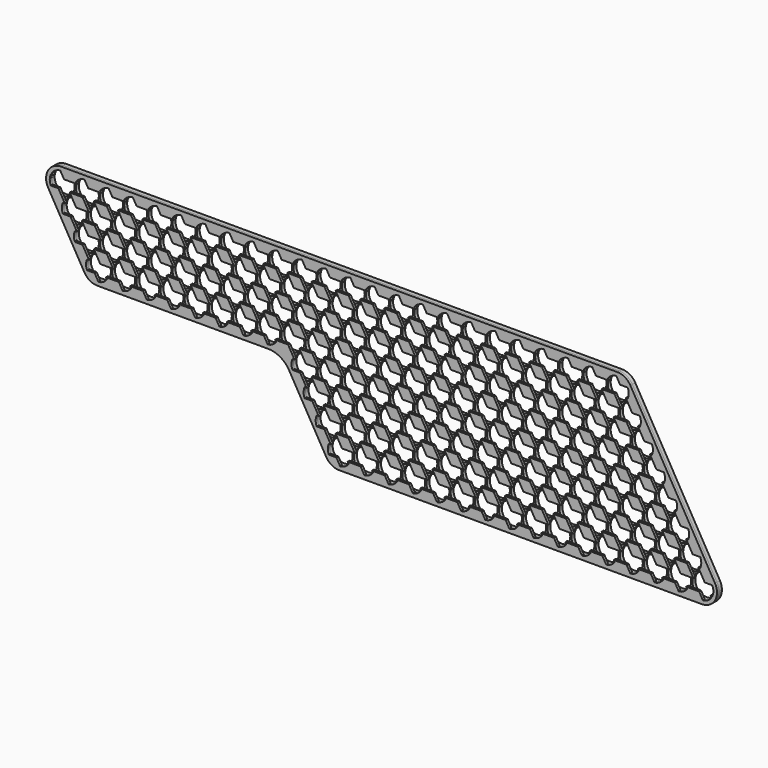
from build123d import *

# Parameters (mm, degrees)
F0_R      = 9.4
F1_DEPTH  = 3
F2_R      = 20
F4_DEPTH  = 2
F6_DEPTH  = 2
F8_DEPTH  = 2
F10_DEPTH = 2
F12_DEPTH = 2


with BuildPart() as f1:
    # F0 (on Front) → F1 (new body)
    with BuildSketch(Plane.XZ):
        with BuildLine():
            ThreePointArc((9.679841755, -7.7498815216), (16.4685048716, -10.4231120583), (19.3, -17.1473029949))
            ThreePointArc((19.3, -17.1473029949), (7.3609322648, -26.1978905469), (1.8716733966, -12.2579296252))
            ThreePointArc((1.8716733966, -12.2579296252), (-5.3694259066, -11.1771760939), (-10.7387150069, -6.2))
            Line((-10.7387150069, -6.2), (18.9612849931, -57.6419089848))
            ThreePointArc((18.9612849931, -57.6419089848), (17.3355686068, -50.5033801767), (20.020158245, -43.6920274632))
            ThreePointArc((20.020158245, -43.6920274632), (13.0758090634, -27.7261011183), (29.2, -34.2946059899))
            ThreePointArc((29.2, -34.2946059899), (28.850587552, -36.833673725), (27.8283266034, -39.1839793596))
            ThreePointArc((27.8283266034, -39.1839793596), (29.7, -39.0419089848), (31.5716733966, -39.1839793596))
            ThreePointArc((31.5716733966, -39.1839793596), (37.0609322648, -25.2440184379), (49, -34.2946059899))
            ThreePointArc((49, -34.2946059899), (46.1685048716, -41.0187969265), (39.379841755, -43.6920274632))
            ThreePointArc((39.379841755, -43.6920274632), (40.4387150069, -45.2419089848), (41.2515151515, -46.9338608812))
            ThreePointArc((41.2515151515, -46.9338608812), (51.8263966154, -42.334336378), (58.9, -51.4419089848))
            ThreePointArc((58.9, -51.4419089848), (51.8263966154, -60.5494815916), (41.2515151515, -55.9499570884))
            ThreePointArc((41.2515151515, -55.9499570884), (36.6950054866, -61.6805562706), (29.7, -63.8419089848))
            Line((29.7, -63.8419089848), (168.3, -63.8419089848))
            ThreePointArc((168.3, -63.8419089848), (161.3049945134, -61.6805562706), (156.7484848485, -55.9499570884))
            ThreePointArc((156.7484848485, -55.9499570884), (139.1, -51.4419089848), (156.7484848485, -46.9338608812))
            ThreePointArc((156.7484848485, -46.9338608812), (157.5612849931, -45.2419089848), (158.620158245, -43.6920274632))
            ThreePointArc((158.620158245, -43.6920274632), (151.6758090634, -27.7261011183), (167.8, -34.2946059899))
            ThreePointArc((167.8, -34.2946059899), (167.450587552, -36.833673725), (166.4283266034, -39.1839793596))
            ThreePointArc((166.4283266034, -39.1839793596), (168.3, -39.0419089848), (170.1716733966, -39.1839793596))
            ThreePointArc((170.1716733966, -39.1839793596), (175.6609322648, -25.2440184379), (187.6, -34.2946059899))
            ThreePointArc((187.6, -34.2946059899), (184.7685048716, -41.0187969265), (177.979841755, -43.6920274632))
            ThreePointArc((177.979841755, -43.6920274632), (179.0387150069, -45.2419089848), (179.8515151515, -46.9338608812))
            ThreePointArc((179.8515151515, -46.9338608812), (190.4263966154, -42.334336378), (197.5, -51.4419089848))
            ThreePointArc((197.5, -51.4419089848), (197.150587552, -53.98097672), (196.1283266034, -56.3312823545))
            ThreePointArc((196.1283266034, -56.3312823545), (198, -56.1892119797), (199.8716733966, -56.3312823545))
            ThreePointArc((199.8716733966, -56.3312823545), (205.3609322648, -42.3913214328), (217.3, -51.4419089848))
            ThreePointArc((217.3, -51.4419089848), (214.4685048716, -58.1660999214), (207.679841755, -60.8393304581))
            ThreePointArc((207.679841755, -60.8393304581), (208.7387150069, -62.3892119797), (209.5515151515, -64.0811638761))
            ThreePointArc((209.5515151515, -64.0811638761), (220.1263966154, -59.4816393729), (227.2, -68.5892119797))
            ThreePointArc((227.2, -68.5892119797), (220.1263966154, -77.6967845865), (209.5515151515, -73.0972600833))
            ThreePointArc((209.5515151515, -73.0972600833), (208.7387150069, -74.7892119797), (207.679841755, -76.3390935013))
            ThreePointArc((207.679841755, -76.3390935013), (214.4685048716, -79.0123240381), (217.3, -85.7365149747))
            ThreePointArc((217.3, -85.7365149747), (205.3609322648, -94.7871025266), (199.8716733966, -80.8471416049))
            ThreePointArc((199.8716733966, -80.8471416049), (192.6305740934, -79.7663880736), (187.2612849931, -74.7892119797))
            Line((187.2612849931, -74.7892119797), (216.9612849931, -126.2311209645))
            ThreePointArc((216.9612849931, -126.2311209645), (215.3355686068, -119.0925921564), (218.020158245, -112.2812394429))
            ThreePointArc((218.020158245, -112.2812394429), (211.0758090634, -96.315313098), (227.2, -102.8838179696))
            ThreePointArc((227.2, -102.8838179696), (226.850587552, -105.4228857048), (225.8283266034, -107.7731913393))
            ThreePointArc((225.8283266034, -107.7731913393), (227.7, -107.6311209645), (229.5716733966, -107.7731913393))
            ThreePointArc((229.5716733966, -107.7731913393), (235.0609322648, -93.8332304176), (247, -102.8838179696))
            ThreePointArc((247, -102.8838179696), (244.1685048716, -109.6080089062), (237.379841755, -112.2812394429))
            ThreePointArc((237.379841755, -112.2812394429), (238.4387150069, -113.8311209645), (239.2515151515, -115.5230728609))
            ThreePointArc((239.2515151515, -115.5230728609), (249.8263966154, -110.9235483577), (256.9, -120.0311209645))
            ThreePointArc((256.9, -120.0311209645), (249.8263966154, -129.1386935713), (239.2515151515, -124.5391690681))
            ThreePointArc((239.2515151515, -124.5391690681), (234.6950054866, -130.2697682503), (227.7, -132.4311209645))
            Line((227.7, -132.4311209645), (524.7, -132.4311209645))
            ThreePointArc((524.7, -132.4311209645), (517.7049945134, -130.2697682503), (513.1484848485, -124.5391690681))
            ThreePointArc((513.1484848485, -124.5391690681), (495.5, -120.0311209645), (513.1484848485, -115.5230728609))
            ThreePointArc((513.1484848485, -115.5230728609), (513.9612849931, -113.8311209645), (515.020158245, -112.2812394429))
            ThreePointArc((515.020158245, -112.2812394429), (508.0758090634, -96.315313098), (524.2, -102.8838179696))
            ThreePointArc((524.2, -102.8838179696), (523.850587552, -105.4228857048), (522.8283266034, -107.7731913393))
            ThreePointArc((522.8283266034, -107.7731913393), (530.0694259066, -108.8539448706), (535.4387150069, -113.8311209645))
            Line((535.4387150069, -113.8311209645), (466.1387150069, 6.2))
            ThreePointArc((466.1387150069, 6.2), (467.377480246, 3.2093561593), (467.8, 0))
            ThreePointArc((467.8, 0), (467.1002144801, -4.1066995409), (465.079841755, -7.7498815216))
            ThreePointArc((465.079841755, -7.7498815216), (471.8685048716, -10.4231120583), (474.7, -17.1473029949))
            ThreePointArc((474.7, -17.1473029949), (462.7609322648, -26.1978905469), (457.2716733966, -12.2579296252))
            ThreePointArc((457.2716733966, -12.2579296252), (455.4, -12.4), (453.5283266034, -12.2579296252))
            ThreePointArc((453.5283266034, -12.2579296252), (454.550587552, -14.6082352597), (454.9, -17.1473029949))
            ThreePointArc((454.9, -17.1473029949), (438.7758090634, -23.7158078665), (445.720158245, -7.7498815216))
            ThreePointArc((445.720158245, -7.7498815216), (444.6612849931, -6.2), (443.8484848485, -4.5080481036))
            ThreePointArc((443.8484848485, -4.5080481036), (426.2, 0), (443.8484848485, 4.5080481036))
            ThreePointArc((443.8484848485, 4.5080481036), (448.4049945134, 10.2386472858), (455.4, 12.4))
            Line((455.4, 12.4), (0, 12.4))
            ThreePointArc((0, 12.4), (6.9950054866, 10.2386472858), (11.5515151515, 4.5080481036))
            ThreePointArc((11.5515151515, 4.5080481036), (22.1263966154, 9.1075726068), (29.2, 0))
            ThreePointArc((29.2, 0), (22.1263966154, -9.1075726068), (11.5515151515, -4.5080481036))
            ThreePointArc((11.5515151515, -4.5080481036), (10.7387150069, -6.2), (9.679841755, -7.7498815216))
        make_face()
        with Locations((257.4, -102.8838179696)):
            Circle(F0_R, mode=Mode.SUBTRACT)
        with Locations((227.7, -85.7365149747)):
            Circle(F0_R, mode=Mode.SUBTRACT)
        with Locations((247.5, -85.7365149747)):
            Circle(F0_R, mode=Mode.SUBTRACT)
        with Locations((237.6, -68.5892119797)):
            Circle(F0_R, mode=Mode.SUBTRACT)
        with Locations((257.4, -68.5892119797)):
            Circle(F0_R, mode=Mode.SUBTRACT)
        with Locations((267.3, -120.0311209645)):
            Circle(F0_R, mode=Mode.SUBTRACT)
        with Locations((287.1, -120.0311209645)):
            Circle(F0_R, mode=Mode.SUBTRACT)
        with Locations((306.9, -120.0311209645)):
            Circle(F0_R, mode=Mode.SUBTRACT)
        with Locations((326.7, -120.0311209645)):
            Circle(F0_R, mode=Mode.SUBTRACT)
        with Locations((346.5, -120.0311209645)):
            Circle(F0_R, mode=Mode.SUBTRACT)
        with Locations((366.3, -120.0311209645)):
            Circle(F0_R, mode=Mode.SUBTRACT)
        with Locations((386.1, -120.0311209645)):
            Circle(F0_R, mode=Mode.SUBTRACT)
        with Locations((277.2, -102.8838179696)):
            Circle(F0_R, mode=Mode.SUBTRACT)
        with Locations((297, -102.8838179696)):
            Circle(F0_R, mode=Mode.SUBTRACT)
        with Locations((316.8, -102.8838179696)):
            Circle(F0_R, mode=Mode.SUBTRACT)
        with Locations((336.6, -102.8838179696)):
            Circle(F0_R, mode=Mode.SUBTRACT)
        with Locations((356.4, -102.8838179696)):
            Circle(F0_R, mode=Mode.SUBTRACT)
        with Locations((376.2, -102.8838179696)):
            Circle(F0_R, mode=Mode.SUBTRACT)
        with Locations((396, -102.8838179696)):
            Circle(F0_R, mode=Mode.SUBTRACT)
        with Locations((405.9, -120.0311209645)):
            Circle(F0_R, mode=Mode.SUBTRACT)
        with Locations((425.7, -120.0311209645)):
            Circle(F0_R, mode=Mode.SUBTRACT)
        with Locations((445.5, -120.0311209645)):
            Circle(F0_R, mode=Mode.SUBTRACT)
        with Locations((465.3, -120.0311209645)):
            Circle(F0_R, mode=Mode.SUBTRACT)
        with Locations((485.1, -120.0311209645)):
            Circle(F0_R, mode=Mode.SUBTRACT)
        with Locations((415.8, -102.8838179696)):
            Circle(F0_R, mode=Mode.SUBTRACT)
        with Locations((435.6, -102.8838179696)):
            Circle(F0_R, mode=Mode.SUBTRACT)
        with Locations((455.4, -102.8838179696)):
            Circle(F0_R, mode=Mode.SUBTRACT)
        with Locations((475.2, -102.8838179696)):
            Circle(F0_R, mode=Mode.SUBTRACT)
        with Locations((495, -102.8838179696)):
            Circle(F0_R, mode=Mode.SUBTRACT)
        with Locations((267.3, -85.7365149747)):
            Circle(F0_R, mode=Mode.SUBTRACT)
        with Locations((287.1, -85.7365149747)):
            Circle(F0_R, mode=Mode.SUBTRACT)
        with Locations((306.9, -85.7365149747)):
            Circle(F0_R, mode=Mode.SUBTRACT)
        with Locations((326.7, -85.7365149747)):
            Circle(F0_R, mode=Mode.SUBTRACT)
        with Locations((346.5, -85.7365149747)):
            Circle(F0_R, mode=Mode.SUBTRACT)
        with Locations((366.3, -85.7365149747)):
            Circle(F0_R, mode=Mode.SUBTRACT)
        with Locations((386.1, -85.7365149747)):
            Circle(F0_R, mode=Mode.SUBTRACT)
        with Locations((277.2, -68.5892119797)):
            Circle(F0_R, mode=Mode.SUBTRACT)
        with Locations((297, -68.5892119797)):
            Circle(F0_R, mode=Mode.SUBTRACT)
        with Locations((316.8, -68.5892119797)):
            Circle(F0_R, mode=Mode.SUBTRACT)
        with Locations((336.6, -68.5892119797)):
            Circle(F0_R, mode=Mode.SUBTRACT)
        with Locations((356.4, -68.5892119797)):
            Circle(F0_R, mode=Mode.SUBTRACT)
        with Locations((376.2, -68.5892119797)):
            Circle(F0_R, mode=Mode.SUBTRACT)
        with Locations((396, -68.5892119797)):
            Circle(F0_R, mode=Mode.SUBTRACT)
        with Locations((405.9, -85.7365149747)):
            Circle(F0_R, mode=Mode.SUBTRACT)
        with Locations((425.7, -85.7365149747)):
            Circle(F0_R, mode=Mode.SUBTRACT)
        with Locations((445.5, -85.7365149747)):
            Circle(F0_R, mode=Mode.SUBTRACT)
        with Locations((465.3, -85.7365149747)):
            Circle(F0_R, mode=Mode.SUBTRACT)
        with Locations((485.1, -85.7365149747)):
            Circle(F0_R, mode=Mode.SUBTRACT)
        with Locations((504.9, -85.7365149747)):
            Circle(F0_R, mode=Mode.SUBTRACT)
        with Locations((415.8, -68.5892119797)):
            Circle(F0_R, mode=Mode.SUBTRACT)
        with Locations((435.6, -68.5892119797)):
            Circle(F0_R, mode=Mode.SUBTRACT)
        with Locations((455.4, -68.5892119797)):
            Circle(F0_R, mode=Mode.SUBTRACT)
        with Locations((475.2, -68.5892119797)):
            Circle(F0_R, mode=Mode.SUBTRACT)
        with Locations((495, -68.5892119797)):
            Circle(F0_R, mode=Mode.SUBTRACT)
        with Locations((69.3, -51.4419089848)):
            Circle(F0_R, mode=Mode.SUBTRACT)
        with Locations((89.1, -51.4419089848)):
            Circle(F0_R, mode=Mode.SUBTRACT)
        with Locations((108.9, -51.4419089848)):
            Circle(F0_R, mode=Mode.SUBTRACT)
        with Locations((59.4, -34.2946059899)):
            Circle(F0_R, mode=Mode.SUBTRACT)
        with Locations((79.2, -34.2946059899)):
            Circle(F0_R, mode=Mode.SUBTRACT)
        with Locations((99, -34.2946059899)):
            Circle(F0_R, mode=Mode.SUBTRACT)
        with Locations((118.8, -34.2946059899)):
            Circle(F0_R, mode=Mode.SUBTRACT)
        with Locations((128.7, -51.4419089848)):
            Circle(F0_R, mode=Mode.SUBTRACT)
        with Locations((227.7, -51.4419089848)):
            Circle(F0_R, mode=Mode.SUBTRACT)
        with Locations((247.5, -51.4419089848)):
            Circle(F0_R, mode=Mode.SUBTRACT)
        with Locations((138.6, -34.2946059899)):
            Circle(F0_R, mode=Mode.SUBTRACT)
        with Locations((198, -34.2946059899)):
            Circle(F0_R, mode=Mode.SUBTRACT)
        with Locations((217.8, -34.2946059899)):
            Circle(F0_R, mode=Mode.SUBTRACT)
        with Locations((237.6, -34.2946059899)):
            Circle(F0_R, mode=Mode.SUBTRACT)
        with Locations((257.4, -34.2946059899)):
            Circle(F0_R, mode=Mode.SUBTRACT)
        with Locations((29.7, -17.1473029949)):
            Circle(F0_R, mode=Mode.SUBTRACT)
        with Locations((49.5, -17.1473029949)):
            Circle(F0_R, mode=Mode.SUBTRACT)
        with Locations((69.3, -17.1473029949)):
            Circle(F0_R, mode=Mode.SUBTRACT)
        with Locations((89.1, -17.1473029949)):
            Circle(F0_R, mode=Mode.SUBTRACT)
        with Locations((108.9, -17.1473029949)):
            Circle(F0_R, mode=Mode.SUBTRACT)
        with Locations((39.6, 0)):
            Circle(F0_R, mode=Mode.SUBTRACT)
        with Locations((59.4, 0)):
            Circle(F0_R, mode=Mode.SUBTRACT)
        with Locations((79.2, 0)):
            Circle(F0_R, mode=Mode.SUBTRACT)
        with Locations((99, 0)):
            Circle(F0_R, mode=Mode.SUBTRACT)
        with Locations((118.8, 0)):
            Circle(F0_R, mode=Mode.SUBTRACT)
        with Locations((128.7, -17.1473029949)):
            Circle(F0_R, mode=Mode.SUBTRACT)
        with Locations((148.5, -17.1473029949)):
            Circle(F0_R, mode=Mode.SUBTRACT)
        with Locations((168.3, -17.1473029949)):
            Circle(F0_R, mode=Mode.SUBTRACT)
        with Locations((188.1, -17.1473029949)):
            Circle(F0_R, mode=Mode.SUBTRACT)
        with Locations((207.9, -17.1473029949)):
            Circle(F0_R, mode=Mode.SUBTRACT)
        with Locations((227.7, -17.1473029949)):
            Circle(F0_R, mode=Mode.SUBTRACT)
        with Locations((247.5, -17.1473029949)):
            Circle(F0_R, mode=Mode.SUBTRACT)
        with Locations((138.6, 0)):
            Circle(F0_R, mode=Mode.SUBTRACT)
        with Locations((158.4, 0)):
            Circle(F0_R, mode=Mode.SUBTRACT)
        with Locations((178.2, 0)):
            Circle(F0_R, mode=Mode.SUBTRACT)
        with Locations((198, 0)):
            Circle(F0_R, mode=Mode.SUBTRACT)
        with Locations((217.8, 0)):
            Circle(F0_R, mode=Mode.SUBTRACT)
        with Locations((237.6, 0)):
            Circle(F0_R, mode=Mode.SUBTRACT)
        with Locations((257.4, 0)):
            Circle(F0_R, mode=Mode.SUBTRACT)
        with Locations((267.3, -51.4419089848)):
            Circle(F0_R, mode=Mode.SUBTRACT)
        with Locations((287.1, -51.4419089848)):
            Circle(F0_R, mode=Mode.SUBTRACT)
        with Locations((306.9, -51.4419089848)):
            Circle(F0_R, mode=Mode.SUBTRACT)
        with Locations((326.7, -51.4419089848)):
            Circle(F0_R, mode=Mode.SUBTRACT)
        with Locations((346.5, -51.4419089848)):
            Circle(F0_R, mode=Mode.SUBTRACT)
        with Locations((366.3, -51.4419089848)):
            Circle(F0_R, mode=Mode.SUBTRACT)
        with Locations((386.1, -51.4419089848)):
            Circle(F0_R, mode=Mode.SUBTRACT)
        with Locations((277.2, -34.2946059899)):
            Circle(F0_R, mode=Mode.SUBTRACT)
        with Locations((297, -34.2946059899)):
            Circle(F0_R, mode=Mode.SUBTRACT)
        with Locations((316.8, -34.2946059899)):
            Circle(F0_R, mode=Mode.SUBTRACT)
        with Locations((336.6, -34.2946059899)):
            Circle(F0_R, mode=Mode.SUBTRACT)
        with Locations((356.4, -34.2946059899)):
            Circle(F0_R, mode=Mode.SUBTRACT)
        with Locations((376.2, -34.2946059899)):
            Circle(F0_R, mode=Mode.SUBTRACT)
        with Locations((396, -34.2946059899)):
            Circle(F0_R, mode=Mode.SUBTRACT)
        with Locations((405.9, -51.4419089848)):
            Circle(F0_R, mode=Mode.SUBTRACT)
        with Locations((425.7, -51.4419089848)):
            Circle(F0_R, mode=Mode.SUBTRACT)
        with Locations((445.5, -51.4419089848)):
            Circle(F0_R, mode=Mode.SUBTRACT)
        with Locations((465.3, -51.4419089848)):
            Circle(F0_R, mode=Mode.SUBTRACT)
        with Locations((485.1, -51.4419089848)):
            Circle(F0_R, mode=Mode.SUBTRACT)
        with Locations((415.8, -34.2946059899)):
            Circle(F0_R, mode=Mode.SUBTRACT)
        with Locations((435.6, -34.2946059899)):
            Circle(F0_R, mode=Mode.SUBTRACT)
        with Locations((455.4, -34.2946059899)):
            Circle(F0_R, mode=Mode.SUBTRACT)
        with Locations((475.2, -34.2946059899)):
            Circle(F0_R, mode=Mode.SUBTRACT)
        with Locations((267.3, -17.1473029949)):
            Circle(F0_R, mode=Mode.SUBTRACT)
        with Locations((287.1, -17.1473029949)):
            Circle(F0_R, mode=Mode.SUBTRACT)
        with Locations((306.9, -17.1473029949)):
            Circle(F0_R, mode=Mode.SUBTRACT)
        with Locations((326.7, -17.1473029949)):
            Circle(F0_R, mode=Mode.SUBTRACT)
        with Locations((346.5, -17.1473029949)):
            Circle(F0_R, mode=Mode.SUBTRACT)
        with Locations((366.3, -17.1473029949)):
            Circle(F0_R, mode=Mode.SUBTRACT)
        with Locations((386.1, -17.1473029949)):
            Circle(F0_R, mode=Mode.SUBTRACT)
        with Locations((277.2, 0)):
            Circle(F0_R, mode=Mode.SUBTRACT)
        with Locations((297, 0)):
            Circle(F0_R, mode=Mode.SUBTRACT)
        with Locations((316.8, 0)):
            Circle(F0_R, mode=Mode.SUBTRACT)
        with Locations((336.6, 0)):
            Circle(F0_R, mode=Mode.SUBTRACT)
        with Locations((356.4, 0)):
            Circle(F0_R, mode=Mode.SUBTRACT)
        with Locations((376.2, 0)):
            Circle(F0_R, mode=Mode.SUBTRACT)
        with Locations((396, 0)):
            Circle(F0_R, mode=Mode.SUBTRACT)
        with Locations((405.9, -17.1473029949)):
            Circle(F0_R, mode=Mode.SUBTRACT)
        with Locations((425.7, -17.1473029949)):
            Circle(F0_R, mode=Mode.SUBTRACT)
        with Locations((415.8, 0)):
            Circle(F0_R, mode=Mode.SUBTRACT)
        with BuildLine():
            ThreePointArc((1.8716733966, -12.2579296252), (5.2, -9.0066641994), (9.679841755, -7.7498815216))
            ThreePointArc((9.679841755, -7.7498815216), (10.7387150069, -6.2), (11.5515151515, -4.5080481036))
            ThreePointArc((11.5515151515, -4.5080481036), (10.4, 0), (11.5515151515, 4.5080481036))
            ThreePointArc((11.5515151515, 4.5080481036), (6.9950054866, 10.2386472858), (0, 12.4))
            ThreePointArc((0, 12.4), (-10.7387150069, 6.2), (-10.7387150069, -6.2))
            ThreePointArc((-10.7387150069, -6.2), (-5.3694259066, -11.1771760939), (1.8716733966, -12.2579296252))
        make_face()
        Circle(F0_R, mode=Mode.SUBTRACT)
        with BuildLine():
            ThreePointArc((20.020158245, -43.6920274632), (17.3355686068, -50.5033801767), (18.9612849931, -57.6419089848))
            ThreePointArc((18.9612849931, -57.6419089848), (23.5, -62.1806239917), (29.7, -63.8419089848))
            ThreePointArc((29.7, -63.8419089848), (36.6950054866, -61.6805562706), (41.2515151515, -55.9499570884))
            ThreePointArc((41.2515151515, -55.9499570884), (40.1, -51.4419089848), (41.2515151515, -46.9338608812))
            ThreePointArc((41.2515151515, -46.9338608812), (40.4387150069, -45.2419089848), (39.379841755, -43.6920274632))
            ThreePointArc((39.379841755, -43.6920274632), (34.9, -42.4352447854), (31.5716733966, -39.1839793596))
            ThreePointArc((31.5716733966, -39.1839793596), (29.7, -39.0419089848), (27.8283266034, -39.1839793596))
            ThreePointArc((27.8283266034, -39.1839793596), (24.5, -42.4352447854), (20.020158245, -43.6920274632))
        make_face()
        with Locations((29.7, -51.4419089848)):
            Circle(F0_R, mode=Mode.SUBTRACT)
        with BuildLine():
            ThreePointArc((466.1387150069, 6.2), (461.6, 10.7387150069), (455.4, 12.4))
            ThreePointArc((455.4, 12.4), (448.4049945134, 10.2386472858), (443.8484848485, 4.5080481036))
            ThreePointArc((443.8484848485, 4.5080481036), (444.7075726068, 2.3263966154), (445, 0))
            ThreePointArc((445, 0), (444.7075726068, -2.3263966154), (443.8484848485, -4.5080481036))
            ThreePointArc((443.8484848485, -4.5080481036), (444.6612849931, -6.2), (445.720158245, -7.7498815216))
            ThreePointArc((445.720158245, -7.7498815216), (450.2, -9.0066641994), (453.5283266034, -12.2579296252))
            ThreePointArc((453.5283266034, -12.2579296252), (455.4, -12.4), (457.2716733966, -12.2579296252))
            ThreePointArc((457.2716733966, -12.2579296252), (460.6, -9.0066641994), (465.079841755, -7.7498815216))
            ThreePointArc((465.079841755, -7.7498815216), (467.1002144801, -4.1066995409), (467.8, 0))
            ThreePointArc((467.8, 0), (467.377480246, 3.2093561593), (466.1387150069, 6.2))
        make_face()
        with Locations((455.4, 0)):
            Circle(F0_R, mode=Mode.SUBTRACT)
        with BuildLine():
            ThreePointArc((156.7484848485, -55.9499570884), (161.3049945134, -61.6805562706), (168.3, -63.8419089848))
            ThreePointArc((168.3, -63.8419089848), (175.2950054866, -61.6805562706), (179.8515151515, -55.9499570884))
            ThreePointArc((179.8515151515, -55.9499570884), (178.7, -51.4419089848), (179.8515151515, -46.9338608812))
            ThreePointArc((179.8515151515, -46.9338608812), (179.0387150069, -45.2419089848), (177.979841755, -43.6920274632))
            ThreePointArc((177.979841755, -43.6920274632), (173.5, -42.4352447854), (170.1716733966, -39.1839793596))
            ThreePointArc((170.1716733966, -39.1839793596), (168.3, -39.0419089848), (166.4283266034, -39.1839793596))
            ThreePointArc((166.4283266034, -39.1839793596), (163.1, -42.4352447854), (158.620158245, -43.6920274632))
            ThreePointArc((158.620158245, -43.6920274632), (157.5612849931, -45.2419089848), (156.7484848485, -46.9338608812))
            ThreePointArc((156.7484848485, -46.9338608812), (157.6075726068, -49.1155123694), (157.9, -51.4419089848))
            ThreePointArc((157.9, -51.4419089848), (157.6075726068, -53.7683056002), (156.7484848485, -55.9499570884))
        make_face()
        with Locations((168.3, -51.4419089848)):
            Circle(F0_R, mode=Mode.SUBTRACT)
        with BuildLine():
            ThreePointArc((179.8515151515, -55.9499570884), (175.2950054866, -61.6805562706), (168.3, -63.8419089848))
            Line((168.3, -63.8419089848), (180.940856662, -63.8419089848))
            Line((180.940856662, -63.8419089848), (187.2612849931, -74.7892119797))
            ThreePointArc((187.2612849931, -74.7892119797), (185.6355686068, -67.6506831716), (188.320158245, -60.8393304581))
            ThreePointArc((188.320158245, -60.8393304581), (183.4, -59.5825477804), (179.8515151515, -55.9499570884))
        make_face()
        with BuildLine():
            ThreePointArc((537.1, -120.0311209645), (536.677480246, -116.8217648053), (535.4387150069, -113.8311209645))
            ThreePointArc((535.4387150069, -113.8311209645), (530.0694259066, -108.8539448706), (522.8283266034, -107.7731913393))
            ThreePointArc((522.8283266034, -107.7731913393), (519.5, -111.0244567652), (515.020158245, -112.2812394429))
            ThreePointArc((515.020158245, -112.2812394429), (513.9612849931, -113.8311209645), (513.1484848485, -115.5230728609))
            ThreePointArc((513.1484848485, -115.5230728609), (514.0075726068, -117.7047243491), (514.3, -120.0311209645))
            ThreePointArc((514.3, -120.0311209645), (514.0075726068, -122.3575175799), (513.1484848485, -124.5391690681))
            ThreePointArc((513.1484848485, -124.5391690681), (517.7049945134, -130.2697682503), (524.7, -132.4311209645))
            ThreePointArc((524.7, -132.4311209645), (533.4681240867, -128.7992450512), (537.1, -120.0311209645))
        make_face()
        with Locations((524.7, -120.0311209645)):
            Circle(F0_R, mode=Mode.SUBTRACT)
        with BuildLine():
            ThreePointArc((196.1283266034, -56.3312823545), (192.8, -59.5825477804), (188.320158245, -60.8393304581))
            ThreePointArc((188.320158245, -60.8393304581), (185.6355686068, -67.6506831716), (187.2612849931, -74.7892119797))
            ThreePointArc((187.2612849931, -74.7892119797), (192.6305740934, -79.7663880736), (199.8716733966, -80.8471416049))
            ThreePointArc((199.8716733966, -80.8471416049), (203.2, -77.5958761791), (207.679841755, -76.3390935013))
            ThreePointArc((207.679841755, -76.3390935013), (208.7387150069, -74.7892119797), (209.5515151515, -73.0972600833))
            ThreePointArc((209.5515151515, -73.0972600833), (208.4, -68.5892119797), (209.5515151515, -64.0811638761))
            ThreePointArc((209.5515151515, -64.0811638761), (208.7387150069, -62.3892119797), (207.679841755, -60.8393304581))
            ThreePointArc((207.679841755, -60.8393304581), (203.2, -59.5825477804), (199.8716733966, -56.3312823545))
            ThreePointArc((199.8716733966, -56.3312823545), (198, -56.1892119797), (196.1283266034, -56.3312823545))
        make_face()
        with Locations((198, -68.5892119797)):
            Circle(F0_R, mode=Mode.SUBTRACT)
        with BuildLine():
            ThreePointArc((218.020158245, -112.2812394429), (215.3355686068, -119.0925921564), (216.9612849931, -126.2311209645))
            ThreePointArc((216.9612849931, -126.2311209645), (221.5, -130.7698359715), (227.7, -132.4311209645))
            ThreePointArc((227.7, -132.4311209645), (234.6950054866, -130.2697682503), (239.2515151515, -124.5391690681))
            ThreePointArc((239.2515151515, -124.5391690681), (238.1, -120.0311209645), (239.2515151515, -115.5230728609))
            ThreePointArc((239.2515151515, -115.5230728609), (238.4387150069, -113.8311209645), (237.379841755, -112.2812394429))
            ThreePointArc((237.379841755, -112.2812394429), (232.9, -111.0244567652), (229.5716733966, -107.7731913393))
            ThreePointArc((229.5716733966, -107.7731913393), (227.7, -107.6311209645), (225.8283266034, -107.7731913393))
            ThreePointArc((225.8283266034, -107.7731913393), (222.5, -111.0244567652), (218.020158245, -112.2812394429))
        make_face()
        with Locations((227.7, -120.0311209645)):
            Circle(F0_R, mode=Mode.SUBTRACT)
    extrude(amount=F1_DEPTH)

    # F2
    f2_edges = [f1.edges().sort_by_distance(p)[0] for p in [
        (180.940857, -1.5, -63.841909),
    ]]
    fillet(f2_edges, radius=F2_R)


with BuildPart() as f4:
    # F3 (on face) → F4 (new body)
    with BuildSketch(Plane.XZ.offset(3)):
        with BuildLine():
            ThreePointArc((466.1387150069, 6.2), (461.6, 10.7387150069), (455.4, 12.4))
            Line((455.4, 12.4), (0, 12.4))
            ThreePointArc((0, 12.4), (-10.7387150069, 6.2), (-10.7387150069, -6.2))
            Line((-10.7387150069, -6.2), (18.9612849931, -57.6419089848))
            ThreePointArc((18.9612849931, -57.6419089848), (23.5, -62.1806239917), (29.7, -63.8419089848))
            Line((29.7, -63.8419089848), (169.3938512783, -63.8419089848))
            ThreePointArc((169.3938512783, -63.8419089848), (179.3938512783, -66.5214009091), (186.7143593539, -73.8419089848))
            Line((186.7143593539, -73.8419089848), (216.9612849931, -126.2311209645))
            ThreePointArc((216.9612849931, -126.2311209645), (221.5, -130.7698359715), (227.7, -132.4311209645))
            Line((227.7, -132.4311209645), (524.7, -132.4311209645))
            ThreePointArc((524.7, -132.4311209645), (535.4387150069, -126.2311209645), (535.4387150069, -113.8311209645))
            Line((535.4387150069, -113.8311209645), (466.1387150069, 6.2))
        make_face()
    extrude(amount=F4_DEPTH)

    # F5 (on face) → F6 (cut, through all)
    with BuildSketch(Plane.XZ.offset(3)):
        with BuildLine():
            Line((0, 4), (-8.5064681273, 4))
            ThreePointArc((-8.5064681273, 4), (-9.4, 0), (-8.5064681273, -4))
            Line((-8.5064681273, -4), (0, -4))
            Line((0, -4), (463.9064681273, -4))
            ThreePointArc((463.9064681273, -4), (464.8, 0), (463.9064681273, 4))
            Line((463.9064681273, 4), (0, 4))
        make_face()
        with BuildLine():
            Line((29.7, -47.4419089848), (21.1935318727, -47.4419089848))
            ThreePointArc((21.1935318727, -47.4419089848), (20.3, -51.4419089848), (21.1935318727, -55.4419089848))
            Line((21.1935318727, -55.4419089848), (29.7, -55.4419089848))
            Line((29.7, -55.4419089848), (493.6064681273, -55.4419089848))
            ThreePointArc((493.6064681273, -55.4419089848), (494.5, -51.4419089848), (493.6064681273, -47.4419089848))
            Line((493.6064681273, -47.4419089848), (29.7, -47.4419089848))
        make_face()
        with BuildLine():
            Line((9.9, -13.1473029949), (1.3935318727, -13.1473029949))
            ThreePointArc((1.3935318727, -13.1473029949), (0.5, -17.1473029949), (1.3935318727, -21.1473029949))
            Line((1.3935318727, -21.1473029949), (9.9, -21.1473029949))
            Line((9.9, -21.1473029949), (473.8064681273, -21.1473029949))
            ThreePointArc((473.8064681273, -21.1473029949), (474.7, -17.1473029949), (473.8064681273, -13.1473029949))
            Line((473.8064681273, -13.1473029949), (9.9, -13.1473029949))
        make_face()
        with BuildLine():
            Line((19.8, -30.2946059899), (11.2935318727, -30.2946059899))
            ThreePointArc((11.2935318727, -30.2946059899), (10.4, -34.2946059899), (11.2935318727, -38.2946059899))
            Line((11.2935318727, -38.2946059899), (19.8, -38.2946059899))
            Line((19.8, -38.2946059899), (483.7064681273, -38.2946059899))
            ThreePointArc((483.7064681273, -38.2946059899), (484.6, -34.2946059899), (483.7064681273, -30.2946059899))
            Line((483.7064681273, -30.2946059899), (19.8, -30.2946059899))
        make_face()
    extrude(amount=F6_DEPTH, mode=Mode.SUBTRACT)

    # F7 (on face) → F8 (cut, through all)
    with BuildSketch(Plane.XZ.offset(3)):
        with BuildLine():
            Line((198, -64.5892119797), (189.4935318727, -64.5892119797))
            ThreePointArc((189.4935318727, -64.5892119797), (188.6, -68.5892119797), (189.4935318727, -72.5892119797))
            Line((189.4935318727, -72.5892119797), (198, -72.5892119797))
            Line((198, -72.5892119797), (495, -72.5892119797))
            Line((495, -72.5892119797), (503.5064681273, -72.5892119797))
            ThreePointArc((503.5064681273, -72.5892119797), (504.4, -68.5892119797), (503.5064681273, -64.5892119797))
            Line((503.5064681273, -64.5892119797), (495, -64.5892119797))
            Line((495, -64.5892119797), (198, -64.5892119797))
        make_face()
        with BuildLine():
            Line((227.7, -116.0311209645), (219.1935318727, -116.0311209645))
            ThreePointArc((219.1935318727, -116.0311209645), (218.3, -120.0311209645), (219.1935318727, -124.0311209645))
            Line((219.1935318727, -124.0311209645), (227.7, -124.0311209645))
            Line((227.7, -124.0311209645), (524.7, -124.0311209645))
            Line((524.7, -124.0311209645), (533.2064681273, -124.0311209645))
            ThreePointArc((533.2064681273, -124.0311209645), (534.1, -120.0311209645), (533.2064681273, -116.0311209645))
            Line((533.2064681273, -116.0311209645), (524.7, -116.0311209645))
            Line((524.7, -116.0311209645), (227.7, -116.0311209645))
        make_face()
        with BuildLine():
            Line((207.9, -81.7365149747), (199.3935318727, -81.7365149747))
            ThreePointArc((199.3935318727, -81.7365149747), (198.5, -85.7365149747), (199.3935318727, -89.7365149747))
            Line((199.3935318727, -89.7365149747), (207.9, -89.7365149747))
            Line((207.9, -89.7365149747), (504.9, -89.7365149747))
            Line((504.9, -89.7365149747), (513.4064681273, -89.7365149747))
            ThreePointArc((513.4064681273, -89.7365149747), (514.3, -85.7365149747), (513.4064681273, -81.7365149747))
            Line((513.4064681273, -81.7365149747), (504.9, -81.7365149747))
            Line((504.9, -81.7365149747), (207.9, -81.7365149747))
        make_face()
        with BuildLine():
            Line((217.8, -98.8838179696), (209.2935318727, -98.8838179696))
            ThreePointArc((209.2935318727, -98.8838179696), (208.4, -102.8838179696), (209.2935318727, -106.8838179696))
            Line((209.2935318727, -106.8838179696), (217.8, -106.8838179696))
            Line((217.8, -106.8838179696), (514.8, -106.8838179696))
            Line((514.8, -106.8838179696), (523.3064681273, -106.8838179696))
            ThreePointArc((523.3064681273, -106.8838179696), (524.2, -102.8838179696), (523.3064681273, -98.8838179696))
            Line((523.3064681273, -98.8838179696), (514.8, -98.8838179696))
            Line((514.8, -98.8838179696), (217.8, -98.8838179696))
        make_face()
    extrude(amount=F8_DEPTH, mode=Mode.SUBTRACT)

    # F9 (on face) → F10 (cut, through all)
    with BuildSketch(Plane.XZ.offset(3)):
        with BuildLine():
            Line((3.4641016151, 2), (-0.7891324485, 9.3668174947))
            ThreePointArc((-0.7891324485, 9.3668174947), (-4.7, 8.1406387956), (-7.7173356788, 5.3668174947))
            Line((-7.7173356788, 5.3668174947), (-3.4641016151, -2))
            Line((-3.4641016151, -2), (26.2358983849, -53.4419089848))
            Line((26.2358983849, -53.4419089848), (30.4891324485, -60.8087264795))
            ThreePointArc((30.4891324485, -60.8087264795), (34.4, -59.5825477804), (37.4173356788, -56.8087264795))
            Line((37.4173356788, -56.8087264795), (33.1641016151, -49.4419089848))
            Line((33.1641016151, -49.4419089848), (3.4641016151, 2))
        make_face()
        with BuildLine():
            Line((23.2641016151, 2), (19.0108675515, 9.3668174947))
            ThreePointArc((19.0108675515, 9.3668174947), (15.1, 8.1406387956), (12.0826643212, 5.3668174947))
            Line((12.0826643212, 5.3668174947), (16.3358983849, -2))
            Line((16.3358983849, -2), (46.0358983849, -53.4419089848))
            Line((46.0358983849, -53.4419089848), (50.2891324485, -60.8087264795))
            ThreePointArc((50.2891324485, -60.8087264795), (54.2, -59.5825477804), (57.2173356788, -56.8087264795))
            Line((57.2173356788, -56.8087264795), (52.9641016151, -49.4419089848))
            Line((52.9641016151, -49.4419089848), (23.2641016151, 2))
        make_face()
        with BuildLine():
            Line((43.0641016151, 2), (38.8108675515, 9.3668174947))
            ThreePointArc((38.8108675515, 9.3668174947), (34.9, 8.1406387956), (31.8826643212, 5.3668174947))
            Line((31.8826643212, 5.3668174947), (36.1358983849, -2))
            Line((36.1358983849, -2), (65.8358983849, -53.4419089848))
            Line((65.8358983849, -53.4419089848), (70.0891324485, -60.8087264795))
            ThreePointArc((70.0891324485, -60.8087264795), (74, -59.5825477804), (77.0173356788, -56.8087264795))
            Line((77.0173356788, -56.8087264795), (72.7641016151, -49.4419089848))
            Line((72.7641016151, -49.4419089848), (43.0641016151, 2))
        make_face()
        with BuildLine():
            Line((62.8641016151, 2), (58.6108675515, 9.3668174947))
            ThreePointArc((58.6108675515, 9.3668174947), (54.7, 8.1406387956), (51.6826643212, 5.3668174947))
            Line((51.6826643212, 5.3668174947), (55.9358983849, -2))
            Line((55.9358983849, -2), (85.6358983849, -53.4419089848))
            Line((85.6358983849, -53.4419089848), (89.8891324485, -60.8087264795))
            ThreePointArc((89.8891324485, -60.8087264795), (93.8, -59.5825477804), (96.8173356788, -56.8087264795))
            Line((96.8173356788, -56.8087264795), (92.5641016151, -49.4419089848))
            Line((92.5641016151, -49.4419089848), (62.8641016151, 2))
        make_face()
        with BuildLine():
            Line((82.6641016151, 2), (78.4108675515, 9.3668174947))
            ThreePointArc((78.4108675515, 9.3668174947), (74.5, 8.1406387956), (71.4826643212, 5.3668174947))
            Line((71.4826643212, 5.3668174947), (75.7358983849, -2))
            Line((75.7358983849, -2), (105.4358983849, -53.4419089848))
            Line((105.4358983849, -53.4419089848), (109.6891324485, -60.8087264795))
            ThreePointArc((109.6891324485, -60.8087264795), (113.6, -59.5825477804), (116.6173356788, -56.8087264795))
            Line((116.6173356788, -56.8087264795), (112.3641016151, -49.4419089848))
            Line((112.3641016151, -49.4419089848), (82.6641016151, 2))
        make_face()
        with BuildLine():
            Line((102.4641016151, 2), (98.2108675515, 9.3668174947))
            ThreePointArc((98.2108675515, 9.3668174947), (94.3, 8.1406387956), (91.2826643212, 5.3668174947))
            Line((91.2826643212, 5.3668174947), (95.5358983849, -2))
            Line((95.5358983849, -2), (125.2358983849, -53.4419089848))
            Line((125.2358983849, -53.4419089848), (129.4891324485, -60.8087264795))
            ThreePointArc((129.4891324485, -60.8087264795), (133.4, -59.5825477804), (136.4173356788, -56.8087264795))
            Line((136.4173356788, -56.8087264795), (132.1641016151, -49.4419089848))
            Line((132.1641016151, -49.4419089848), (102.4641016151, 2))
        make_face()
        with BuildLine():
            Line((122.2641016151, 2), (118.0108675515, 9.3668174947))
            ThreePointArc((118.0108675515, 9.3668174947), (114.1, 8.1406387956), (111.0826643212, 5.3668174947))
            Line((111.0826643212, 5.3668174947), (115.3358983849, -2))
            Line((115.3358983849, -2), (145.0358983849, -53.4419089848))
            Line((145.0358983849, -53.4419089848), (149.2891324485, -60.8087264795))
            ThreePointArc((149.2891324485, -60.8087264795), (153.2, -59.5825477804), (156.2173356788, -56.8087264795))
            Line((156.2173356788, -56.8087264795), (151.9641016151, -49.4419089848))
            Line((151.9641016151, -49.4419089848), (122.2641016151, 2))
        make_face()
        with BuildLine():
            Line((142.0641016151, 2), (137.8108675515, 9.3668174947))
            ThreePointArc((137.8108675515, 9.3668174947), (133.9, 8.1406387956), (130.8826643212, 5.3668174947))
            Line((130.8826643212, 5.3668174947), (135.1358983849, -2))
            Line((135.1358983849, -2), (164.8358983849, -53.4419089848))
            Line((164.8358983849, -53.4419089848), (169.0891324485, -60.8087264795))
            ThreePointArc((169.0891324485, -60.8087264795), (173, -59.5825477804), (176.0173356788, -56.8087264795))
            Line((176.0173356788, -56.8087264795), (171.7641016151, -49.4419089848))
            Line((171.7641016151, -49.4419089848), (142.0641016151, 2))
        make_face()
    extrude(amount=F10_DEPTH, mode=Mode.SUBTRACT)

    # F11 (on face) → F12 (cut, through all)
    with BuildSketch(Plane.XZ.offset(3)):
        with BuildLine():
            Line((161.8641016151, 2), (157.6108675515, 9.3668174947))
            ThreePointArc((157.6108675515, 9.3668174947), (153.7, 8.1406387956), (150.6826643212, 5.3668174947))
            Line((150.6826643212, 5.3668174947), (154.9358983849, -2))
            Line((154.9358983849, -2), (224.2358983849, -122.0311209645))
            Line((224.2358983849, -122.0311209645), (228.4891324485, -129.3979384592))
            ThreePointArc((228.4891324485, -129.3979384592), (232.4, -128.1717597601), (235.4173356788, -125.3979384592))
            Line((235.4173356788, -125.3979384592), (231.1641016151, -118.0311209645))
            Line((231.1641016151, -118.0311209645), (161.8641016151, 2))
        make_face()
        with BuildLine():
            Line((181.6641016151, 2), (177.4108675515, 9.3668174947))
            ThreePointArc((177.4108675515, 9.3668174947), (173.5, 8.1406387956), (170.4826643212, 5.3668174947))
            Line((170.4826643212, 5.3668174947), (174.7358983849, -2))
            Line((174.7358983849, -2), (244.0358983849, -122.0311209645))
            Line((244.0358983849, -122.0311209645), (248.2891324485, -129.3979384592))
            ThreePointArc((248.2891324485, -129.3979384592), (252.2, -128.1717597601), (255.2173356788, -125.3979384592))
            Line((255.2173356788, -125.3979384592), (250.9641016151, -118.0311209645))
            Line((250.9641016151, -118.0311209645), (181.6641016151, 2))
        make_face()
        with BuildLine():
            Line((201.4641016151, 2), (197.2108675515, 9.3668174947))
            ThreePointArc((197.2108675515, 9.3668174947), (193.3, 8.1406387956), (190.2826643212, 5.3668174947))
            Line((190.2826643212, 5.3668174947), (194.5358983849, -2))
            Line((194.5358983849, -2), (263.8358983849, -122.0311209645))
            Line((263.8358983849, -122.0311209645), (268.0891324485, -129.3979384592))
            ThreePointArc((268.0891324485, -129.3979384592), (272, -128.1717597601), (275.0173356788, -125.3979384592))
            Line((275.0173356788, -125.3979384592), (270.7641016151, -118.0311209645))
            Line((270.7641016151, -118.0311209645), (201.4641016151, 2))
        make_face()
        with BuildLine():
            Line((221.2641016151, 2), (217.0108675515, 9.3668174947))
            ThreePointArc((217.0108675515, 9.3668174947), (213.1, 8.1406387956), (210.0826643212, 5.3668174947))
            Line((210.0826643212, 5.3668174947), (214.3358983849, -2))
            Line((214.3358983849, -2), (283.6358983849, -122.0311209645))
            Line((283.6358983849, -122.0311209645), (287.8891324485, -129.3979384592))
            ThreePointArc((287.8891324485, -129.3979384592), (291.8, -128.1717597601), (294.8173356788, -125.3979384592))
            Line((294.8173356788, -125.3979384592), (290.5641016151, -118.0311209645))
            Line((290.5641016151, -118.0311209645), (221.2641016151, 2))
        make_face()
        with BuildLine():
            Line((241.0641016151, 2), (236.8108675515, 9.3668174947))
            ThreePointArc((236.8108675515, 9.3668174947), (232.9, 8.1406387956), (229.8826643212, 5.3668174947))
            Line((229.8826643212, 5.3668174947), (234.1358983849, -2))
            Line((234.1358983849, -2), (303.4358983849, -122.0311209645))
            Line((303.4358983849, -122.0311209645), (307.6891324485, -129.3979384592))
            ThreePointArc((307.6891324485, -129.3979384592), (311.6, -128.1717597601), (314.6173356788, -125.3979384592))
            Line((314.6173356788, -125.3979384592), (310.3641016151, -118.0311209645))
            Line((310.3641016151, -118.0311209645), (241.0641016151, 2))
        make_face()
        with BuildLine():
            Line((260.8641016151, 2), (256.6108675515, 9.3668174947))
            ThreePointArc((256.6108675515, 9.3668174947), (252.7, 8.1406387956), (249.6826643212, 5.3668174947))
            Line((249.6826643212, 5.3668174947), (253.9358983849, -2))
            Line((253.9358983849, -2), (323.2358983849, -122.0311209645))
            Line((323.2358983849, -122.0311209645), (327.4891324485, -129.3979384592))
            ThreePointArc((327.4891324485, -129.3979384592), (331.4, -128.1717597601), (334.4173356788, -125.3979384592))
            Line((334.4173356788, -125.3979384592), (330.1641016151, -118.0311209645))
            Line((330.1641016151, -118.0311209645), (260.8641016151, 2))
        make_face()
        with BuildLine():
            Line((280.6641016151, 2), (276.4108675515, 9.3668174947))
            ThreePointArc((276.4108675515, 9.3668174947), (272.5, 8.1406387956), (269.4826643212, 5.3668174947))
            Line((269.4826643212, 5.3668174947), (273.7358983849, -2))
            Line((273.7358983849, -2), (343.0358983849, -122.0311209645))
            Line((343.0358983849, -122.0311209645), (347.2891324485, -129.3979384592))
            ThreePointArc((347.2891324485, -129.3979384592), (351.2, -128.1717597601), (354.2173356788, -125.3979384592))
            Line((354.2173356788, -125.3979384592), (349.9641016151, -118.0311209645))
            Line((349.9641016151, -118.0311209645), (280.6641016151, 2))
        make_face()
        with BuildLine():
            Line((300.4641016151, 2), (296.2108675515, 9.3668174947))
            ThreePointArc((296.2108675515, 9.3668174947), (292.3, 8.1406387956), (289.2826643212, 5.3668174947))
            Line((289.2826643212, 5.3668174947), (293.5358983849, -2))
            Line((293.5358983849, -2), (362.8358983849, -122.0311209645))
            Line((362.8358983849, -122.0311209645), (367.0891324485, -129.3979384592))
            ThreePointArc((367.0891324485, -129.3979384592), (371, -128.1717597601), (374.0173356788, -125.3979384592))
            Line((374.0173356788, -125.3979384592), (369.7641016151, -118.0311209645))
            Line((369.7641016151, -118.0311209645), (300.4641016151, 2))
        make_face()
        with BuildLine():
            Line((320.2641016151, 2), (316.0108675515, 9.3668174947))
            ThreePointArc((316.0108675515, 9.3668174947), (312.1, 8.1406387956), (309.0826643212, 5.3668174947))
            Line((309.0826643212, 5.3668174947), (313.3358983849, -2))
            Line((313.3358983849, -2), (382.6358983849, -122.0311209645))
            Line((382.6358983849, -122.0311209645), (386.8891324485, -129.3979384592))
            ThreePointArc((386.8891324485, -129.3979384592), (390.8, -128.1717597601), (393.8173356788, -125.3979384592))
            Line((393.8173356788, -125.3979384592), (389.5641016151, -118.0311209645))
            Line((389.5641016151, -118.0311209645), (320.2641016151, 2))
        make_face()
        with BuildLine():
            Line((340.0641016151, 2), (335.8108675515, 9.3668174947))
            ThreePointArc((335.8108675515, 9.3668174947), (331.9, 8.1406387956), (328.8826643212, 5.3668174947))
            Line((328.8826643212, 5.3668174947), (333.1358983849, -2))
            Line((333.1358983849, -2), (402.4358983849, -122.0311209645))
            Line((402.4358983849, -122.0311209645), (406.6891324485, -129.3979384592))
            ThreePointArc((406.6891324485, -129.3979384592), (410.6, -128.1717597601), (413.6173356788, -125.3979384592))
            Line((413.6173356788, -125.3979384592), (409.3641016151, -118.0311209645))
            Line((409.3641016151, -118.0311209645), (340.0641016151, 2))
        make_face()
        with BuildLine():
            Line((359.8641016151, 2), (355.6108675515, 9.3668174947))
            ThreePointArc((355.6108675515, 9.3668174947), (351.7, 8.1406387956), (348.6826643212, 5.3668174947))
            Line((348.6826643212, 5.3668174947), (352.9358983849, -2))
            Line((352.9358983849, -2), (422.2358983849, -122.0311209645))
            Line((422.2358983849, -122.0311209645), (426.4891324485, -129.3979384592))
            ThreePointArc((426.4891324485, -129.3979384592), (430.4, -128.1717597601), (433.4173356788, -125.3979384592))
            Line((433.4173356788, -125.3979384592), (429.1641016151, -118.0311209645))
            Line((429.1641016151, -118.0311209645), (359.8641016151, 2))
        make_face()
        with BuildLine():
            Line((379.6641016151, 2), (375.4108675515, 9.3668174947))
            ThreePointArc((375.4108675515, 9.3668174947), (371.5, 8.1406387956), (368.4826643212, 5.3668174947))
            Line((368.4826643212, 5.3668174947), (372.7358983849, -2))
            Line((372.7358983849, -2), (442.0358983849, -122.0311209645))
            Line((442.0358983849, -122.0311209645), (446.2891324485, -129.3979384592))
            ThreePointArc((446.2891324485, -129.3979384592), (450.2, -128.1717597601), (453.2173356788, -125.3979384592))
            Line((453.2173356788, -125.3979384592), (448.9641016151, -118.0311209645))
            Line((448.9641016151, -118.0311209645), (379.6641016151, 2))
        make_face()
        with BuildLine():
            Line((399.4641016151, 2), (395.2108675515, 9.3668174947))
            ThreePointArc((395.2108675515, 9.3668174947), (391.3, 8.1406387956), (388.2826643212, 5.3668174947))
            Line((388.2826643212, 5.3668174947), (392.5358983849, -2))
            Line((392.5358983849, -2), (461.8358983849, -122.0311209645))
            Line((461.8358983849, -122.0311209645), (466.0891324485, -129.3979384592))
            ThreePointArc((466.0891324485, -129.3979384592), (470, -128.1717597601), (473.0173356788, -125.3979384592))
            Line((473.0173356788, -125.3979384592), (468.7641016151, -118.0311209645))
            Line((468.7641016151, -118.0311209645), (399.4641016151, 2))
        make_face()
        with BuildLine():
            Line((419.2641016151, 2), (415.0108675515, 9.3668174947))
            ThreePointArc((415.0108675515, 9.3668174947), (411.1, 8.1406387956), (408.0826643212, 5.3668174947))
            Line((408.0826643212, 5.3668174947), (412.3358983849, -2))
            Line((412.3358983849, -2), (481.6358983849, -122.0311209645))
            Line((481.6358983849, -122.0311209645), (485.8891324485, -129.3979384592))
            ThreePointArc((485.8891324485, -129.3979384592), (489.8, -128.1717597601), (492.8173356788, -125.3979384592))
            Line((492.8173356788, -125.3979384592), (488.5641016151, -118.0311209645))
            Line((488.5641016151, -118.0311209645), (419.2641016151, 2))
        make_face()
        with BuildLine():
            Line((439.0641016151, 2), (434.8108675515, 9.3668174947))
            ThreePointArc((434.8108675515, 9.3668174947), (430.9, 8.1406387956), (427.8826643212, 5.3668174947))
            Line((427.8826643212, 5.3668174947), (432.1358983849, -2))
            Line((432.1358983849, -2), (501.4358983849, -122.0311209645))
            Line((501.4358983849, -122.0311209645), (505.6891324485, -129.3979384592))
            ThreePointArc((505.6891324485, -129.3979384592), (509.6, -128.1717597601), (512.6173356788, -125.3979384592))
            Line((512.6173356788, -125.3979384592), (508.3641016151, -118.0311209645))
            Line((508.3641016151, -118.0311209645), (439.0641016151, 2))
        make_face()
        with BuildLine():
            Line((458.8641016151, 2), (454.6108675515, 9.3668174947))
            ThreePointArc((454.6108675515, 9.3668174947), (450.7, 8.1406387956), (447.6826643212, 5.3668174947))
            Line((447.6826643212, 5.3668174947), (451.9358983849, -2))
            Line((451.9358983849, -2), (521.2358983849, -122.0311209645))
            Line((521.2358983849, -122.0311209645), (525.4891324485, -129.3979384592))
            ThreePointArc((525.4891324485, -129.3979384592), (529.4, -128.1717597601), (532.4173356788, -125.3979384592))
            Line((532.4173356788, -125.3979384592), (528.1641016151, -118.0311209645))
            Line((528.1641016151, -118.0311209645), (458.8641016151, 2))
        make_face()
    extrude(amount=F12_DEPTH, mode=Mode.SUBTRACT)


solid = Compound([f1.part, f4.part])
